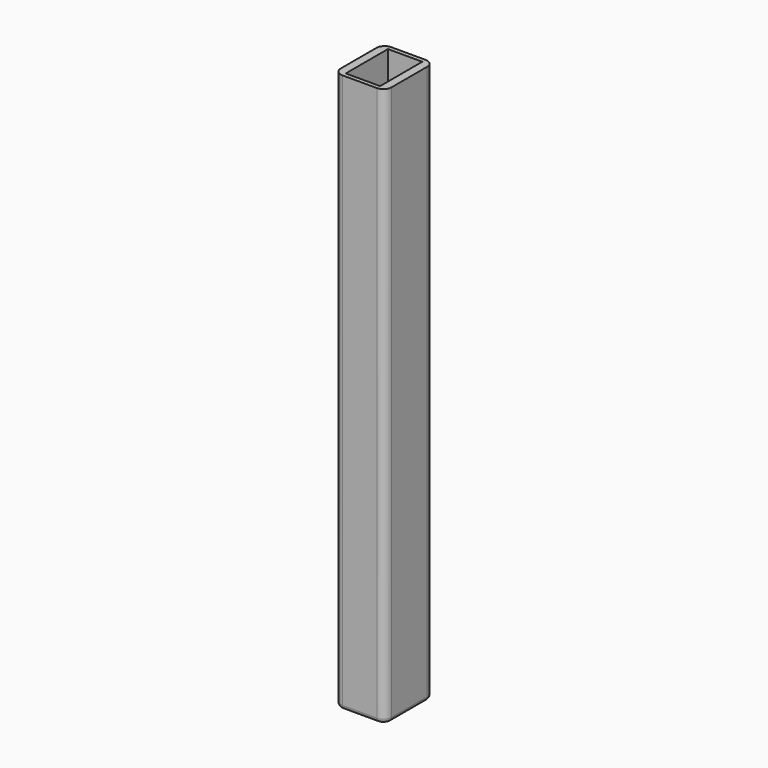
from build123d import *

# Parameters (mm, degrees)
F0_W         = 24.6
F0_H         = 29.5
F0_W_2       = 16.6
F0_H_2       = 25.5
F1_DEPTH     = 270
F2_R         = 1.99999
F3_T1_DEPTH  = 280
F3_T4_ANGLE  = 90
F3_T6_ANGLE  = 90
F3_T8_ANGLE  = 90
F3_T10_ANGLE = 90


# Not quite as in the source:
# - a fillet or chamfer that OpenCascade refuses, or shapes differently, is made with other operations: its cross-section is extruded or revolved along the edge and cut away or added
# - a fillet or chamfer is up to 0.001 mm smaller than in the source, because OpenCascade refuses the exact size


with BuildPart() as f1:
    # F0 (on Top) → F1 (new body)
    with BuildSketch(Plane.XY):
        Rectangle(F0_W, F0_H)
        Rectangle(F0_W_2, F0_H_2, mode=Mode.SUBTRACT)
    extrude(amount=-F1_DEPTH)

    # F2 (radius 2 in the source; OpenCascade refuses exactly that, so slightly less here)
    f2_edges = [f1.edges().sort_by_distance(p)[0] for p in [
        (-12.3, 0, -270),
        (0, 14.75, -270),
        (12.3, 0, -270),
        (0, -14.75, -270),
    ]]
    fillet(f2_edges, radius=F2_R)

    # F3: fillet of radius 4 on 4 edges, made by hand

    # F3_s2 → F3_t1 (cut)
    with BuildSketch(Plane.XY.offset(-270)):
        with BuildLine():
            ThreePointArc((8.3, 14.75), (11.1284271247, 13.5784271247), (12.3, 10.75))
            Line((12.3, 10.75), (12.3, 14.75))
            Line((12.3, 14.75), (8.3, 14.75))
        make_face()
        with BuildLine():
            ThreePointArc((-12.3, 10.75), (-11.1284271247, 13.5784271247), (-8.3, 14.75))
            Line((-8.3, 14.75), (-12.3, 14.75))
            Line((-12.3, 14.75), (-12.3, 10.75))
        make_face()
        with BuildLine():
            ThreePointArc((8.3, -14.75), (11.1284271247, -13.5784271247), (12.3, -10.75))
            Line((12.3, -10.75), (12.3, -14.75))
            Line((12.3, -14.75), (8.3, -14.75))
        make_face()
        with BuildLine():
            ThreePointArc((-12.3, -10.75), (-11.1284271247, -13.5784271247), (-8.3, -14.75))
            Line((-8.3, -14.75), (-12.3, -14.75))
            Line((-12.3, -14.75), (-12.3, -10.75))
        make_face()
    extrude(amount=F3_T1_DEPTH, mode=Mode.SUBTRACT)

    # F3_s3 → F3_t4 (revolve, cut)
    with BuildSketch(Plane.YZ.offset(-8.3)):
        with BuildLine():
            ThreePointArc((-12.75001, -270), (-14.1642164913, -269.4142164913), (-14.75, -268.00001))
            Line((-14.75, -268.00001), (-14.75, -270))
            Line((-14.75, -270), (-12.75001, -270))
        make_face()
    revolve(axis=Axis((-8.3, -10.75, -270), (0, 0, -1)), revolution_arc=F3_T4_ANGLE, mode=Mode.SUBTRACT)

    # F3_s5 → F3_t6 (revolve, cut)
    with BuildSketch(Plane.XZ.offset(10.75)):
        with BuildLine():
            ThreePointArc((10.30001, -270), (11.7142164913, -269.4142164913), (12.3, -268.00001))
            Line((12.3, -268.00001), (12.3, -270))
            Line((12.3, -270), (10.30001, -270))
        make_face()
    revolve(axis=Axis((8.3, -10.75, -270), (0, 0, -1)), revolution_arc=F3_T6_ANGLE, mode=Mode.SUBTRACT)

    # F3_s7 → F3_t8 (revolve, cut)
    with BuildSketch(Plane.XZ.offset(-10.75)):
        with BuildLine():
            ThreePointArc((-10.30001, -270), (-11.7142164913, -269.4142164913), (-12.3, -268.00001))
            Line((-12.3, -268.00001), (-12.3, -270))
            Line((-12.3, -270), (-10.30001, -270))
        make_face()
    revolve(axis=Axis((-8.3, 10.75, -270), (0, 0, -1)), revolution_arc=F3_T8_ANGLE, mode=Mode.SUBTRACT)

    # F3_s9 → F3_t10 (revolve, cut)
    with BuildSketch(Plane.YZ.offset(8.3)):
        with BuildLine():
            ThreePointArc((12.75001, -270), (14.1642164913, -269.4142164913), (14.75, -268.00001))
            Line((14.75, -268.00001), (14.75, -270))
            Line((14.75, -270), (12.75001, -270))
        make_face()
    revolve(axis=Axis((8.3, 10.75, -270), (0, 0, -1)), revolution_arc=F3_T10_ANGLE, mode=Mode.SUBTRACT)


solid = f1.part
